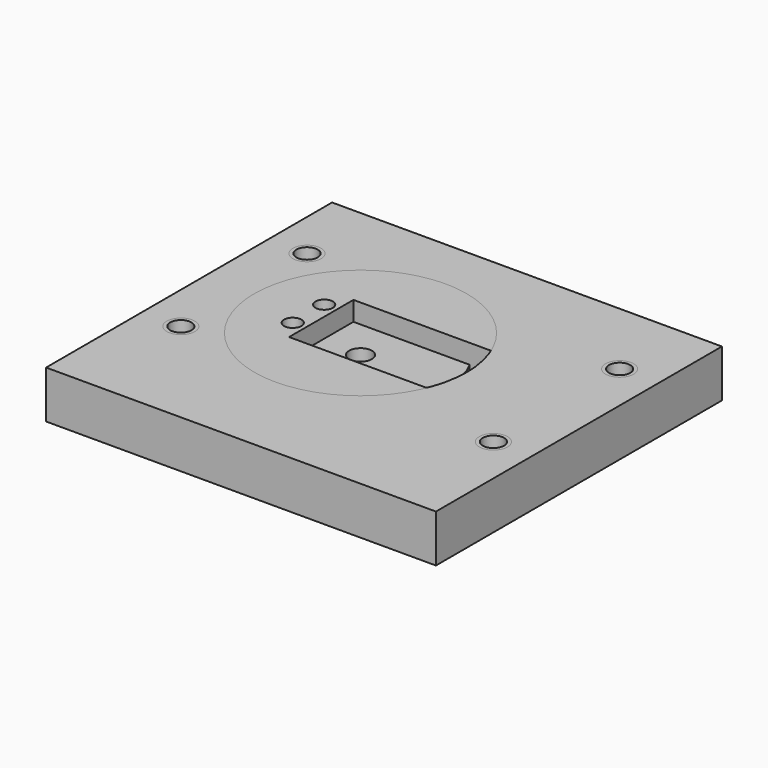
from build123d import *
from build123d import SkipClean  # not in build123d's __all__

# Parameters (mm, degrees)
F1_W           = 100.88
F1_H           = 60.82
F1_W_2         = 40.88
F1_H_2         = 20.82
F2_DEPTH       = 9.5
F3_D           = 4.5
F4_D           = 5.5
F5_W           = 100.88
F5_H           = 92.5
F5_R           = 2.95
F6_DEPTH       = 12.3
F7_DEPTH       = 10
F8_DEPTH       = 5
F9_D           = 5.5
F9_CBORE_D     = 7.3
F9_CBORE_DEPTH = 5


with BuildPart() as f2:
    # F1 (on Top) → F2 (new body)
    with BuildSketch(Plane.XY):
        Rectangle(F1_W, F1_H)
        Rectangle(F1_W_2, F1_H_2, mode=Mode.SUBTRACT)
    extrude(amount=-F2_DEPTH)

    # F3 (through all)
    with Locations(Plane.XY):
        with Locations((-23.75, 5.085), (-23.75, -5.085), (23.51, -5.085), (23.51, 5.085), (23.51, -5.085)):
            Hole(F3_D / 2)

    # F4 (through all)
    with Locations(Plane.XY):
        with Locations((-40.44, 20.41), (-40.44, -20.41), (40.44, -20.41), (40.44, 20.41)):
            Hole(F4_D / 2)


with BuildPart() as f6:
    # F5 (on Top) → F6 (new body)
    with BuildSketch(Plane.XY):
        with Locations((0, -5.25)):
            Rectangle(F5_W, F5_H)
        with BuildLine():
            ThreePointArc((-7.33, 27.3413148916), (9.1654364826, 19.4454364826), (17.0613148916, 2.95))
            ThreePointArc((17.0613148916, 2.95), (17.1803000668, 1.4771324385), (17.22, 0))
            ThreePointArc((17.22, 0), (17.1803000668, -1.4771324385), (17.0613148916, -2.95))
            ThreePointArc((17.0613148916, -2.95), (9.1654364826, -19.4454364826), (-7.33, -27.3413148916))
            ThreePointArc((-7.33, -27.3413148916), (-10.28, -27.5), (-13.23, -27.3413148916))
            ThreePointArc((-13.23, -27.3413148916), (-29.7254364826, -19.4454364826), (-37.6213148916, -2.95))
            ThreePointArc((-37.6213148916, -2.95), (-37.78, 0), (-37.6213148916, 2.95))
            ThreePointArc((-37.6213148916, 2.95), (-29.7254364826, 19.4454364826), (-13.23, 27.3413148916))
            ThreePointArc((-13.23, 27.3413148916), (-10.28, 27.5), (-7.33, 27.3413148916))
        make_face(mode=Mode.SUBTRACT)
        with BuildLine():
            ThreePointArc((-32.5857727954, -2.95), (-32.78, 0), (-32.5857727954, 2.95))
            Line((-32.5857727954, 2.95), (-37.6213148916, 2.95))
            ThreePointArc((-37.6213148916, 2.95), (-37.78, 0), (-37.6213148916, -2.95))
            Line((-37.6213148916, -2.95), (-32.5857727954, -2.95))
        make_face()
        with BuildLine():
            ThreePointArc((12.0257727954, -2.95), (12.1713906907, -1.4781935096), (12.22, 0))
            ThreePointArc((12.22, 0), (12.1713906907, 1.4781935096), (12.0257727954, 2.95))
            ThreePointArc((12.0257727954, 2.95), (5.6299025767, 15.9099025767), (-7.33, 22.3057727954))
            ThreePointArc((-7.33, 22.3057727954), (-10.28, 22.5), (-13.23, 22.3057727954))
            ThreePointArc((-13.23, 22.3057727954), (-26.1899025767, 15.9099025767), (-32.5857727954, 2.95))
            ThreePointArc((-32.5857727954, 2.95), (-32.78, 0), (-32.5857727954, -2.95))
            ThreePointArc((-32.5857727954, -2.95), (-26.1899025767, -15.9099025767), (-13.23, -22.3057727954))
            ThreePointArc((-13.23, -22.3057727954), (-10.28, -22.5), (-7.33, -22.3057727954))
            ThreePointArc((-7.33, -22.3057727954), (5.6299025767, -15.9099025767), (12.0257727954, -2.95))
        make_face()
        with Locations((-10.28, 0)):
            Circle(F5_R, mode=Mode.SUBTRACT)
        with BuildLine():
            ThreePointArc((-13.23, 22.3057727954), (-10.28, 22.5), (-7.33, 22.3057727954))
            Line((-7.33, 22.3057727954), (-7.33, 27.3413148916))
            ThreePointArc((-7.33, 27.3413148916), (-10.28, 27.5), (-13.23, 27.3413148916))
            Line((-13.23, 27.3413148916), (-13.23, 22.3057727954))
        make_face()
        with BuildLine():
            ThreePointArc((12.0257727954, 2.95), (12.1713906907, 1.4781935096), (12.22, 0))
            ThreePointArc((12.22, 0), (12.1713906907, -1.4781935096), (12.0257727954, -2.95))
            Line((12.0257727954, -2.95), (17.0613148916, -2.95))
            ThreePointArc((17.0613148916, -2.95), (17.1803000668, -1.4771324385), (17.22, 0))
            ThreePointArc((17.22, 0), (17.1803000668, 1.4771324385), (17.0613148916, 2.95))
            Line((17.0613148916, 2.95), (12.0257727954, 2.95))
        make_face()
        with BuildLine():
            Line((-7.33, -27.3413148916), (-7.33, -22.3057727954))
            ThreePointArc((-7.33, -22.3057727954), (-10.28, -22.5), (-13.23, -22.3057727954))
            Line((-13.23, -22.3057727954), (-13.23, -27.3413148916))
            ThreePointArc((-13.23, -27.3413148916), (-10.28, -27.5), (-7.33, -27.3413148916))
        make_face()
    extrude(amount=-F6_DEPTH)

    # F5 (on Top) → F7 (cut)
    with BuildSketch(Plane.XY):
        with BuildLine():
            ThreePointArc((-13.23, 22.3057727954), (-10.28, 22.5), (-7.33, 22.3057727954))
            Line((-7.33, 22.3057727954), (-7.33, 27.3413148916))
            ThreePointArc((-7.33, 27.3413148916), (-10.28, 27.5), (-13.23, 27.3413148916))
            Line((-13.23, 27.3413148916), (-13.23, 22.3057727954))
        make_face()
        with BuildLine():
            ThreePointArc((-32.5857727954, -2.95), (-32.78, 0), (-32.5857727954, 2.95))
            Line((-32.5857727954, 2.95), (-37.6213148916, 2.95))
            ThreePointArc((-37.6213148916, 2.95), (-37.78, 0), (-37.6213148916, -2.95))
            Line((-37.6213148916, -2.95), (-32.5857727954, -2.95))
        make_face()
        with BuildLine():
            Line((-7.33, -27.3413148916), (-7.33, -22.3057727954))
            ThreePointArc((-7.33, -22.3057727954), (-10.28, -22.5), (-13.23, -22.3057727954))
            Line((-13.23, -22.3057727954), (-13.23, -27.3413148916))
            ThreePointArc((-13.23, -27.3413148916), (-10.28, -27.5), (-7.33, -27.3413148916))
        make_face()
        with BuildLine():
            ThreePointArc((12.0257727954, 2.95), (12.1713906907, 1.4781935096), (12.22, 0))
            ThreePointArc((12.22, 0), (12.1713906907, -1.4781935096), (12.0257727954, -2.95))
            Line((12.0257727954, -2.95), (17.0613148916, -2.95))
            ThreePointArc((17.0613148916, -2.95), (17.1803000668, -1.4771324385), (17.22, 0))
            ThreePointArc((17.22, 0), (17.1803000668, 1.4771324385), (17.0613148916, 2.95))
            Line((17.0613148916, 2.95), (12.0257727954, 2.95))
        make_face()
    with SkipClean():  # cleaning this boolean's faces spoils the solid; the shape is the same uncleaned
        extrude(amount=-F7_DEPTH, mode=Mode.SUBTRACT)

    # F5 (on Top) → F8 (cut)
    with BuildSketch(Plane.XY):
        with BuildLine():
            ThreePointArc((12.0257727954, -2.95), (12.1713906907, -1.4781935096), (12.22, 0))
            ThreePointArc((12.22, 0), (12.1713906907, 1.4781935096), (12.0257727954, 2.95))
            ThreePointArc((12.0257727954, 2.95), (5.6299025767, 15.9099025767), (-7.33, 22.3057727954))
            ThreePointArc((-7.33, 22.3057727954), (-10.28, 22.5), (-13.23, 22.3057727954))
            ThreePointArc((-13.23, 22.3057727954), (-26.1899025767, 15.9099025767), (-32.5857727954, 2.95))
            ThreePointArc((-32.5857727954, 2.95), (-32.78, 0), (-32.5857727954, -2.95))
            ThreePointArc((-32.5857727954, -2.95), (-26.1899025767, -15.9099025767), (-13.23, -22.3057727954))
            ThreePointArc((-13.23, -22.3057727954), (-10.28, -22.5), (-7.33, -22.3057727954))
            ThreePointArc((-7.33, -22.3057727954), (5.6299025767, -15.9099025767), (12.0257727954, -2.95))
        make_face()
        with Locations((-10.28, 0)):
            Circle(F5_R, mode=Mode.SUBTRACT)
    extrude(amount=-F8_DEPTH, mode=Mode.SUBTRACT)

    # F9 (through all)
    with Locations(Plane.XY):
        with Locations((-40.44, 20.41), (-40.44, -20.41), (40.44, -20.41), (40.44, 20.41)):
            CounterBoreHole(F9_D / 2, F9_CBORE_D / 2, F9_CBORE_DEPTH)


solid = Compound([f2.part, f6.part])
